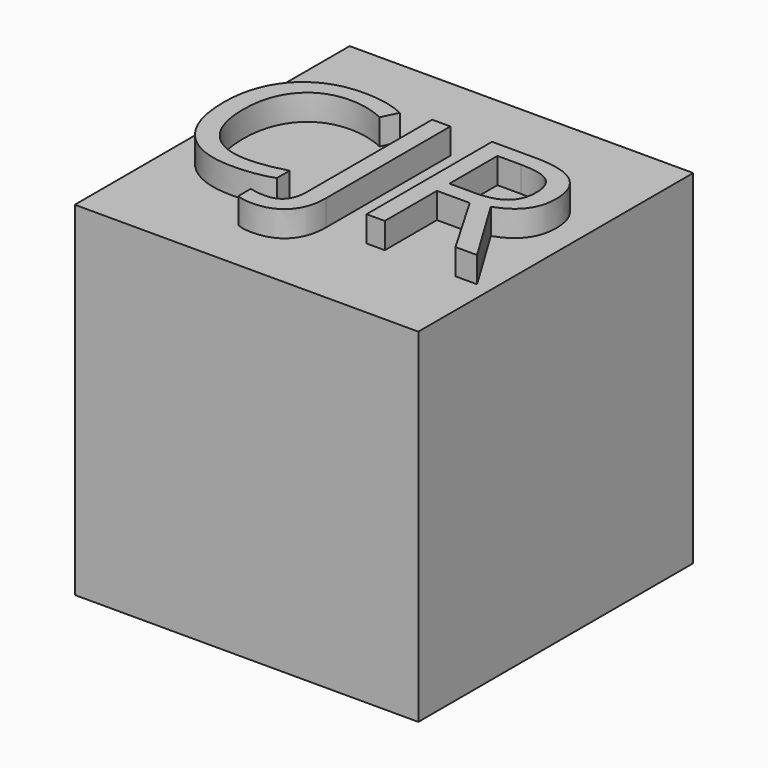
from build123d import *

# Parameters (mm, degrees)
F0_W         = 40
F0_H         = 40
F1_DEPTH     = 40
F2_TEXT_SIZE = 25.5769807174
F3_DEPTH     = 3


# Not quite as in the source:
# - Text() gives the source's letters only with a copy of the font that has no kerning and outlines rounded to 1/6400 em; it was checked with that copy


with BuildPart() as f1:
    # F0 (on Front) → F1 (new body)
    with BuildSketch(Plane.XZ):
        with Locations((20, 20)):
            Rectangle(F0_W, F0_H)
    extrude(amount=-F1_DEPTH)

    # F2 (on face) → F3 (join)
    with BuildSketch(Plane.XY.offset(40)):
        with Locations((0, 10.6119640084)):
            Text('CJR', F2_TEXT_SIZE, font='Open Sans', text_align=(TextAlign.LEFT, TextAlign.BOTTOM))
    extrude(amount=F3_DEPTH)


solid = f1.part
